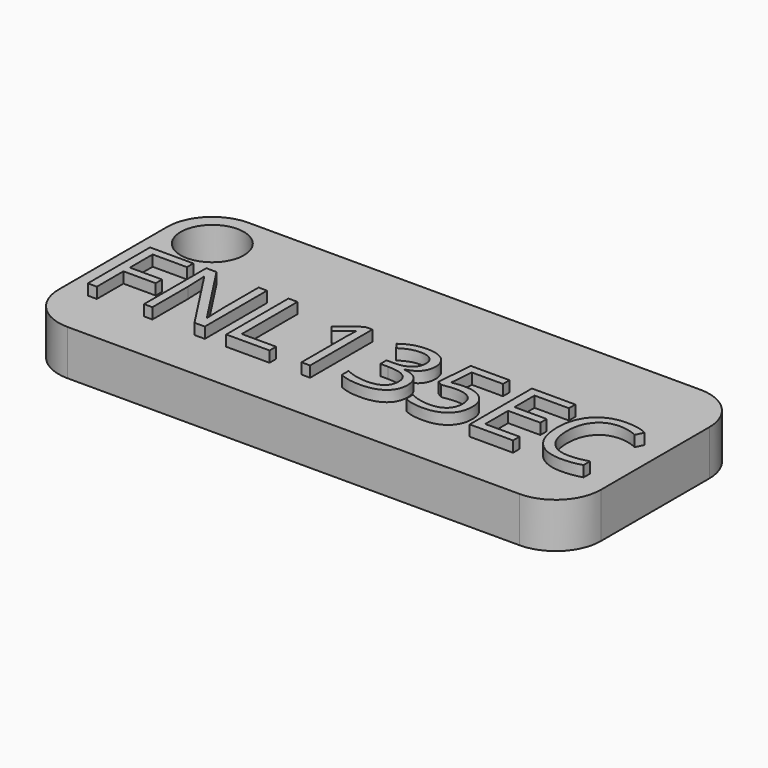
from build123d import *

# Parameters (mm, degrees)
F0_W         = 60
F0_H         = 25
F1_DEPTH     = 5
F3_D         = 7
F4_R         = 5
F5_TEXT_SIZE = 12.0603015075
F6_DEPTH     = 1.2


# Not quite as in the source:
# - Text() gives the source's letters only with a copy of the font that has no kerning and outlines rounded to 1/6400 em; it was checked with that copy


with BuildPart() as f1:
    # F0 (on Top) → F1 (new body)
    with BuildSketch(Plane.XY):
        Rectangle(F0_W, F0_H)
    extrude(amount=F1_DEPTH)

    # F3 (through all)
    with Locations(Plane.XY.offset(5)):
        with Locations((-25, 7.500000298)):
            Hole(F3_D / 2)

    # F4
    f4_edges = [f1.edges().sort_by_distance(p)[0] for p in [
        (30, -12.5, 2.5),
        (-30, -12.5, 2.5),
        (-30, 12.5, 2.5),
        (30, 12.5, 2.5),
    ]]
    fillet(f4_edges, radius=F4_R)

    # F5 (on face) → F6 (join)
    with BuildSketch(Plane.XY.offset(5)):
        with Locations((-28.5, -6.8280687013)):
            Text('FNL135EC', F5_TEXT_SIZE, font='Open Sans', text_align=(TextAlign.LEFT, TextAlign.BOTTOM))
    extrude(amount=F6_DEPTH)


solid = f1.part
